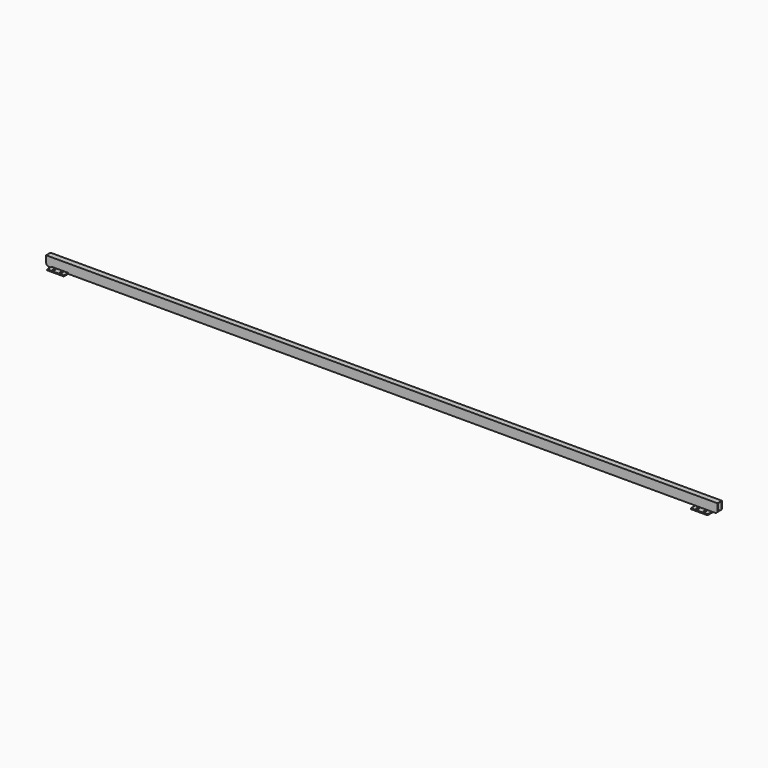
from build123d import *

# Parameters (mm, degrees)
F0_W          = 3575
F0_H          = 50
F1_DEPTH      = 15
F1_DEPTH_BACK = 15
F3_DEPTH      = 5
F5_DEPTH      = 5
F6_R          = 6
F7_DEPTH      = 5
F8_R          = 6
F9_DEPTH      = 5
F12_DEPTH     = 5
F13_W         = 30
F13_H         = 50
F14_DEPTH     = 30
F15_R         = 15
F16_W         = 26
F16_H         = 13
F16_H_2       = 33
F17_DEPTH     = 100
F18_W         = 30
F18_H         = 50
F19_DEPTH     = 30
F20_W         = 26
F20_H         = 46
F21_DEPTH     = 100
F22_T1_DEPTH  = 105
F23_DEPTH     = 5
F24_DEPTH     = 5


# Not quite as in the source:
# - a fillet or chamfer that OpenCascade refuses, or shapes differently, is made with other operations: its cross-section is extruded or revolved along the edge and cut away or added


with BuildPart() as f1:
    # F0 (on Front) → F1 (new body, two sides)
    with BuildSketch(Plane.XZ) as f1_sk:
        Rectangle(F0_W, F0_H)
    extrude(amount=F1_DEPTH)
    extrude(f1_sk.sketch, amount=-F1_DEPTH_BACK)

    # F2 (on face) → F3 (join)
    with BuildSketch(Plane(origin=(0, 0, -25), x_dir=(1, 0, 0), z_dir=(0, 0, -1))):
        Polygon((-1787.5, 45), (-1787.5, 15), (-1787.5, -15), (-1697.5, -15), (-1697.5, 45), align=None)
    extrude(amount=F3_DEPTH)

    # F4 (on face) → F5 (join)
    with BuildSketch(Plane(origin=(0, 0, -25), x_dir=(1, 0, 0), z_dir=(0, 0, -1))):
        Polygon((1787.5, -15), (1787.5, 15), (1787.5, 45), (1697.5, 45), (1697.5, -15), align=None)
    extrude(amount=F5_DEPTH)

    # F6 (on face) → F7 (cut, through all)
    with BuildSketch(Plane(origin=(0, 0, -30), x_dir=(1, 0, 0), z_dir=(0, 0, -1))):
        with Locations((-935, 30)):
            Circle(F6_R)
        with Locations((-975, 30)):
            Circle(F6_R)
    extrude(amount=-F7_DEPTH, mode=Mode.SUBTRACT)

    # F8 (on face) → F9 (cut, through all)
    with BuildSketch(Plane(origin=(0, 0, -30), x_dir=(1, 0, 0), z_dir=(0, 0, -1))):
        with Locations((1762.5, 30)):
            Circle(F8_R)
        with Locations((1722.5, 30)):
            Circle(F8_R)
    extrude(amount=-F9_DEPTH, mode=Mode.SUBTRACT)

    # F11 (on face) → F12 (cut, through all)
    with BuildSketch(Plane(origin=(0, 0, -30), x_dir=(1, 0, 0), z_dir=(0, 0, -1))):
        with BuildLine():
            ThreePointArc((-1762.5, 36), (-1766.7426406871, 34.2426406871), (-1768.5, 30))
            Line((-1768.5, 30), (-1762.5, 30))
            Line((-1762.5, 30), (-1762.5, 36))
        make_face()
        with BuildLine():
            ThreePointArc((-1716.5, 30), (-1722.5, 36), (-1728.5, 30))
            ThreePointArc((-1728.5, 30), (-1722.5, 24), (-1716.5, 30))
        make_face()
        with BuildLine():
            Line((-1762.5, 30), (-1768.5, 30))
            ThreePointArc((-1768.5, 30), (-1762.5, 24), (-1756.5, 30))
            Line((-1756.5, 30), (-1762.5, 30))
        make_face()
        with BuildLine():
            Line((-1762.5, 36), (-1762.5, 30))
            Line((-1762.5, 30), (-1756.5, 30))
            ThreePointArc((-1756.5, 30), (-1758.2573593129, 34.2426406871), (-1762.5, 36))
        make_face()
    extrude(amount=-F12_DEPTH, mode=Mode.SUBTRACT)

    # F13 (on face) → F14 (join)
    with BuildSketch(Plane.YZ.offset(1787.5)):
        Rectangle(F13_W, F13_H)
    extrude(amount=F14_DEPTH)

    # F15
    f15_edges = [f1.edges().sort_by_distance(p)[0] for p in [
        (1817.5, 0, -25),
    ]]
    fillet(f15_edges, radius=F15_R)

    # F16 (on face) → F17 (cut)
    with BuildSketch(Plane.YZ.offset(1817.5)):
        with Locations((0, -16.5)):
            Rectangle(F16_W, F16_H)
        with Locations((0, 6.5)):
            Rectangle(F16_W, F16_H_2)
    extrude(amount=-F17_DEPTH, mode=Mode.SUBTRACT)

    # F18 (on face) → F19 (join)
    with BuildSketch(Plane(origin=(-1787.5, 0, 0), x_dir=(0, -1, 0), z_dir=(-1, 0, 0))):
        Rectangle(F18_W, F18_H)
    extrude(amount=F19_DEPTH)

    # F20 (on face) → F21 (cut)
    with BuildSketch(Plane(origin=(-1817.5, 0, 0), x_dir=(0, -1, 0), z_dir=(-1, 0, 0))):
        Rectangle(F20_W, F20_H)
    extrude(amount=-F21_DEPTH, mode=Mode.SUBTRACT)

    # F22: fillet of radius 15 on 1 edges, made by hand

    # F22_s2 → F22_t1 (cut)
    with BuildSketch(Plane.XZ.offset(-52.5)):
        with BuildLine():
            ThreePointArc((-1817.5, -10), (-1813.1066017178, -20.6066017178), (-1802.5, -25))
            Line((-1802.5, -25), (-1817.5, -25))
            Line((-1817.5, -25), (-1817.5, -10))
        make_face()
    extrude(amount=F22_T1_DEPTH, mode=Mode.SUBTRACT)

    # F23 (add): a face of the model
    f23_faces = [f1.faces().sort_by_distance(p)[0] for p in [
        (-1742.5, -30, -25),
    ]]
    extrude(f23_faces, amount=F23_DEPTH)

    # F24 (cut): a face of the model
    f24_faces = [f1.faces().sort_by_distance(p)[0] for p in [
        (-1742.5, -14.3442118808, -30),
    ]]
    extrude(f24_faces, amount=-F24_DEPTH, mode=Mode.SUBTRACT)


solid = f1.part
